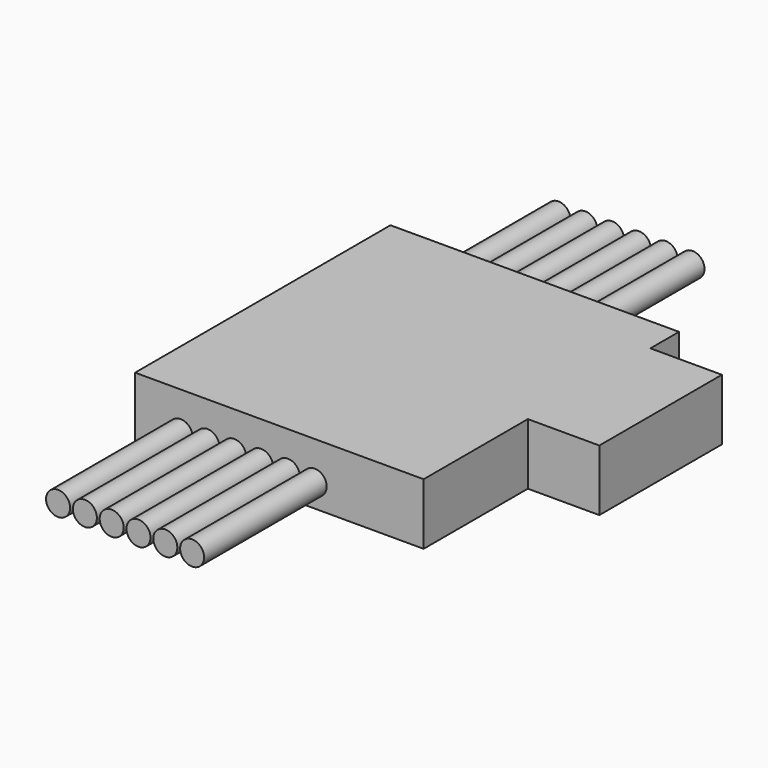
from build123d import *

# Parameters (mm, degrees)
F0_W     = 56.5
F0_H     = 62.5
F1_DEPTH = 12
F2_R     = 2.35
F3_DEPTH = 30
F4_R     = 2.35
F5_DEPTH = 30
F7_DEPTH = 14
F9_DEPTH = 0.1


with BuildPart() as f1:
    # F0 (on Top) → F1 (new body)
    with BuildSketch(Plane.XY):
        Rectangle(F0_W, F0_H)
    extrude(amount=F1_DEPTH)

    # F2 (on face) → F3 (join)
    with BuildSketch(Plane.XZ.offset(31.25)):
        with Locations((-19.333169, 4.546953)):
            Circle(F2_R)
        with Locations((-14.083169, 4.546953)):
            Circle(F2_R)
        with Locations((-8.833169, 4.546953)):
            Circle(F2_R)
        with Locations((-3.583169, 4.546953)):
            Circle(F2_R)
        with Locations((1.666831, 4.546953)):
            Circle(F2_R)
        with Locations((6.916831, 4.546953)):
            Circle(F2_R)
    extrude(amount=F3_DEPTH)

    # F4 (on face) → F5 (join)
    with BuildSketch(Plane(origin=(0, 31.25, 0), x_dir=(-1, 0, 0), z_dir=(0, 1, 0))):
        with Locations((-6.8952, 4.455985)):
            Circle(F4_R)
        with Locations((-1.6452, 4.455985)):
            Circle(F4_R)
        with Locations((3.6048, 4.455985)):
            Circle(F4_R)
        with Locations((8.8548, 4.455985)):
            Circle(F4_R)
        with Locations((14.1048, 4.455985)):
            Circle(F4_R)
        with Locations((19.3548, 4.455985)):
            Circle(F4_R)
    extrude(amount=F5_DEPTH)

    # F6 (on face) → F7 (join)
    with BuildSketch(Plane.YZ.offset(28.25)):
        Polygon((24.25, 0), (24.25, 6), (24.25, 12), (-5.75, 12), (-5.75, 0), align=None)
    extrude(amount=F7_DEPTH)

    # F8 (on face) → F9 (join)
    with BuildSketch(Plane(origin=(0, 0, 0), x_dir=(1, 0, 0), z_dir=(0, 0, -1))):
        Polygon((-23.225292, 21.77481), (-25.547083, 21.77481), (-24.398697, 10.295952), (-21.481446, 10.295952), (-15.494326, 21.77481), (-17.996257, 21.77481), (-19.339793, 19.05271), (-23.037647, 19.05271), align=None)
        with BuildLine():
            Line((-22.7174, 14.28403), (-22.920056, 17.021142))
            Line((-22.920056, 17.021142), (-20.318048, 17.021142))
            Line((-20.318048, 17.021142), (-21.786681, 14.011319))
            add(Edge.make_bspline(
                [(-22.63984, 12.024787), (-22.294573, 12.963011), (-21.786681, 14.011319)],
                knots=[0, 0, 0, 1, 1, 1], degree=2))
            Line((-22.63984, 12.024787), (-22.63984, 12.307505))
            add(Edge.make_bspline(
                [(-22.7174, 14.28403), (-22.63984, 13.26074), (-22.63984, 12.307505)],
                knots=[0, 0, 0, 1, 1, 1], degree=2))
        make_face(mode=Mode.SUBTRACT)
        with BuildLine():
            Line((-10.168231, 21.77481), (-12.500607, 21.77481))
            add(Edge.make_bspline(
                [(-14.997693, 19.734486), (-14.033181, 21.343837), (-12.500607, 21.77481)],
                knots=[0, 0, 0, 0.732207, 0.732207, 0.732207], degree=2))
            add(Edge.make_bspline(
                [(-16.314959, 13.861204), (-16.314959, 17.53654), (-14.997693, 19.734486)],
                knots=[0, 0, 0, 1, 1, 1], degree=2))
            add(Edge.make_bspline(
                [(-13.195052, 10.16335), (-16.314959, 10.16335), (-16.314959, 13.861204)],
                knots=[0, 0, 0, 1, 1, 1], degree=2))
            add(Edge.make_bspline(
                [(-10.590542, 11.105327), (-11.716411, 10.16335), (-13.195052, 10.16335)],
                knots=[0, 0, 0, 1, 1, 1], degree=2))
            add(Edge.make_bspline(
                [(-8.807916, 13.923752), (-9.464673, 12.047304), (-10.590542, 11.105327)],
                knots=[0, 0, 0, 1, 1, 1], degree=2))
            add(Edge.make_bspline(
                [(-8.151159, 18.124493), (-8.151159, 15.8002), (-8.807916, 13.923752)],
                knots=[0, 0, 0, 1, 1, 1], degree=2))
            add(Edge.make_bspline(
                [(-8.953028, 20.977945), (-8.151159, 20.023459), (-8.151159, 18.124493)],
                knots=[0, 0, 0, 1, 1, 1], degree=2))
            add(Edge.make_bspline(
                [(-10.168231, 21.77481), (-9.429041, 21.544556), (-8.953028, 20.977945)],
                knots=[0.406371, 0.406371, 0.406371, 1, 1, 1], degree=2))
        make_face()
        with BuildLine():
            add(Edge.make_bspline(
                [(-12.984889, 12.11986), (-12.359407, 12.11986), (-11.815237, 12.932987)],
                knots=[0, 0, 0, 1, 1, 1], degree=2))
            add(Edge.make_bspline(
                [(-13.706696, 12.517667), (-13.467762, 12.11986), (-12.984889, 12.11986)],
                knots=[0, 0, 0, 1, 1, 1], degree=2))
            add(Edge.make_bspline(
                [(-13.945631, 13.783644), (-13.945631, 12.915474), (-13.706696, 12.517667)],
                knots=[0, 0, 0, 1, 1, 1], degree=2))
            add(Edge.make_bspline(
                [(-13.5816, 16.802223), (-13.945631, 15.277296), (-13.945631, 13.783644)],
                knots=[0, 0, 0, 1, 1, 1], degree=2))
            add(Edge.make_bspline(
                [(-12.67465, 19.155289), (-13.217569, 18.32715), (-13.5816, 16.802223)],
                knots=[0, 0, 0, 1, 1, 1], degree=2))
            add(Edge.make_bspline(
                [(-11.498743, 19.983428), (-12.131731, 19.983428), (-12.67465, 19.155289)],
                knots=[0, 0, 0, 1, 1, 1], degree=2))
            add(Edge.make_bspline(
                [(-10.735654, 19.526826), (-10.95082, 19.983428), (-11.498743, 19.983428)],
                knots=[0, 0, 0, 1, 1, 1], degree=2))
            add(Edge.make_bspline(
                [(-10.520488, 18.169528), (-10.520488, 19.070223), (-10.735654, 19.526826)],
                knots=[0, 0, 0, 1, 1, 1], degree=2))
            add(Edge.make_bspline(
                [(-10.895777, 15.293559), (-10.520488, 16.841003), (-10.520488, 18.169528)],
                knots=[0, 0, 0, 1, 1, 1], degree=2))
            add(Edge.make_bspline(
                [(-11.815237, 12.932987), (-11.271067, 13.746115), (-10.895777, 15.293559)],
                knots=[0, 0, 0, 1, 1, 1], degree=2))
        make_face(mode=Mode.SUBTRACT)
        with BuildLine():
            Line((1.566339, 21.77481), (-5.954464, 21.77481))
            Line((-5.954464, 21.77481), (-6.377291, 19.740741))
            Line((-6.377291, 19.740741), (-1.936364, 19.740741))
            Line((-1.936364, 19.740741), (-1.936364, 19.663181))
            Line((-1.936364, 19.663181), (-4.040487, 17.926841))
            add(Edge.make_bspline(
                [(-6.123345, 16.012864), (-5.486603, 16.748432), (-4.040487, 17.926841)],
                knots=[0, 0, 0, 1, 1, 1], degree=2))
            add(Edge.make_bspline(
                [(-7.080333, 14.54298), (-6.760086, 15.277296), (-6.123345, 16.012864)],
                knots=[0, 0, 0, 1, 1, 1], degree=2))
            add(Edge.make_bspline(
                [(-7.40058, 12.970516), (-7.40058, 13.808663), (-7.080333, 14.54298)],
                knots=[0, 0, 0, 1, 1, 1], degree=2))
            add(Edge.make_bspline(
                [(-6.533661, 10.946454), (-7.40058, 11.712045), (-7.40058, 12.970516)],
                knots=[0, 0, 0, 1, 1, 1], degree=2))
            add(Edge.make_bspline(
                [(-4.180596, 10.180864), (-5.666742, 10.180864), (-6.533661, 10.946454)],
                knots=[0, 0, 0, 1, 1, 1], degree=2))
            add(Edge.make_bspline(
                [(-2.226588, 10.551149), (-3.164812, 10.180864), (-4.180596, 10.180864)],
                knots=[0, 0, 0, 1, 1, 1], degree=2))
            add(Edge.make_bspline(
                [(-0.255066, 11.797111), (-1.288364, 10.921435), (-2.226588, 10.551149)],
                knots=[0, 0, 0, 1, 1, 1], degree=2))
            Line((-0.255066, 11.797111), (-1.395947, 13.385837))
            add(Edge.make_bspline(
                [(-2.736982, 12.458871), (-2.194063, 12.720323), (-1.395947, 13.385837)],
                knots=[0, 0, 0, 1, 1, 1], degree=2))
            add(Edge.make_bspline(
                [(-3.7978, 12.19742), (-3.279901, 12.19742), (-2.736982, 12.458871)],
                knots=[0, 0, 0, 1, 1, 1], degree=2))
            add(Edge.make_bspline(
                [(-4.657213, 12.506408), (-4.335715, 12.19742), (-3.7978, 12.19742)],
                knots=[0, 0, 0, 1, 1, 1], degree=2))
            add(Edge.make_bspline(
                [(-4.978711, 13.400848), (-4.978711, 12.815397), (-4.657213, 12.506408)],
                knots=[0, 0, 0, 1, 1, 1], degree=2))
            add(Edge.make_bspline(
                [(-4.442047, 14.804431), (-4.978711, 14.058856), (-4.978711, 13.400848)],
                knots=[0, 0, 0, 1, 1, 1], degree=2))
            add(Edge.make_bspline(
                [(-2.499298, 16.793466), (-3.905383, 15.550007), (-4.442047, 14.804431)],
                knots=[0, 0, 0, 1, 1, 1], degree=2))
            Line((-2.499298, 16.793466), (1.23108, 20.108524))
            Line((1.23108, 20.108524), (1.566339, 21.77481))
        make_face()
        Polygon((6.720316, 17.293852), (10.465706, 21.77481), (7.728594, 21.77481), (5.664501, 19.100246), (4.686247, 21.77481), (2.136779, 21.77481), (4.045752, 17.418949), (0.392934, 13.033065), (3.162571, 13.033065), (5.069042, 15.64508), (5.969737, 13.033065), (8.479173, 13.033065), align=None)
        Polygon((14.083498, 19.405482), (14.576378, 21.77481), (12.287112, 21.77481), (11.794232, 19.405482), (10.463204, 19.405482), (10.065397, 17.529034), (11.393923, 17.529034), (9.870247, 10.343489), (12.302123, 10.343489), (18.321769, 17.576571), (18.697058, 19.405482), align=None)
        with BuildLine():
            Line((13.232842, 15.590038), (13.685691, 17.529034))
            Line((13.685691, 17.529034), (16.117568, 17.529034))
            Line((16.117568, 17.529034), (13.67068, 14.621791))
            add(Edge.make_bspline(
                [(12.637382, 13.205698), (12.912595, 13.698578), (13.67068, 14.621791)],
                knots=[0, 0, 0, 1, 1, 1], degree=2))
            Line((12.637382, 13.205698), (12.589845, 13.205698))
            add(Edge.make_bspline(
                [(12.918849, 14.307798), (12.69993, 13.478408), (12.589845, 13.205698)],
                knots=[0, 0, 0, 1, 1, 1], degree=2))
            add(Edge.make_bspline(
                [(13.232842, 15.590038), (13.137768, 15.137188), (12.918849, 14.307798)],
                knots=[0, 0, 0, 1, 1, 1], degree=2))
        make_face(mode=Mode.SUBTRACT)
    extrude(amount=F9_DEPTH)


solid = f1.part
